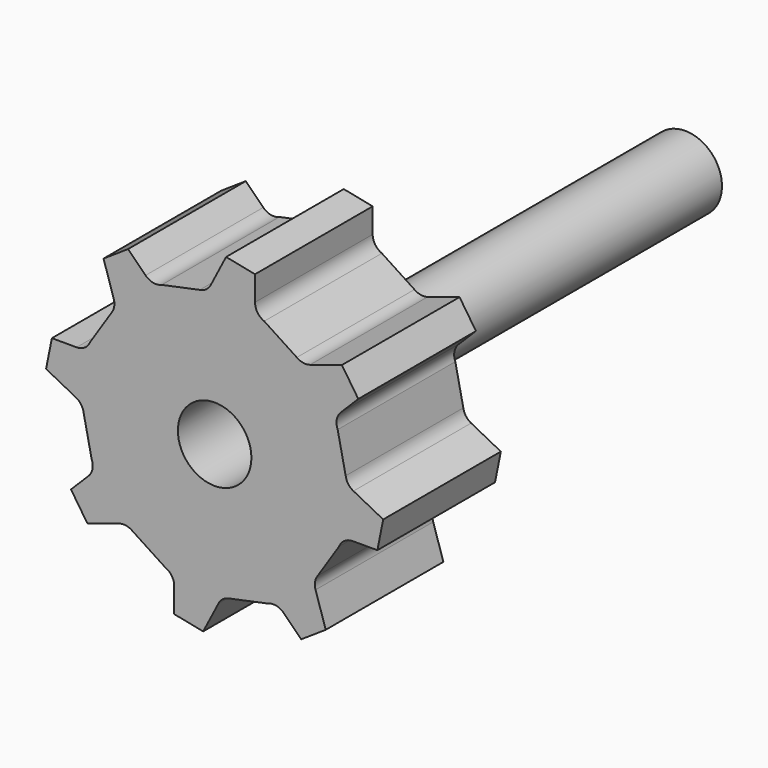
from build123d import *

# Parameters (mm, degrees)
F0_R     = 12.5
F1_DEPTH = 50
F2_R     = 12.5
F3_DEPTH = 150


with BuildPart() as f1:
    # F0 (on Front) → F1 (new body)
    with BuildSketch(Plane.XZ):
        with BuildLine():
            Line((-116.0371901115, -128.3445464136), (-125.8805584276, -126.3758683266))
            Line((-125.8805584276, -126.3758683266), (-131.1020102552, -136.4806844073))
            ThreePointArc((-131.1020102552, -136.4806844073), (-132.6345582421, -138.2516897117), (-134.8054626168, -139.1305169507))
            Line((-134.8054626168, -139.1305169507), (-147.7560899978, -141.8494963995))
            ThreePointArc((-147.7560899978, -141.8494963995), (-150.6647489323, -142.156192832), (-153.2473327671, -140.7833781193))
            Line((-153.2473327671, -140.7833781193), (-159.1905657596, -134.8401451268))
            Line((-159.1905657596, -134.8401451268), (-167.5429438709, -140.4083919875))
            Line((-167.5429438709, -140.4083919875), (-164.0898838925, -151.2456999557))
            ThreePointArc((-164.0898838925, -151.2456999557), (-163.9212691063, -153.5816648901), (-164.8349056108, -155.738150795))
            Line((-164.8349056108, -155.738150795), (-172.0697732464, -166.8182360428))
            ThreePointArc((-172.0697732464, -166.8182360428), (-173.9096385759, -169.0918356267), (-176.7065277112, -169.9472715767))
            Line((-176.7065277112, -169.9472715767), (-185.1115284135, -169.9472715767))
            Line((-185.1115284135, -169.9472715767), (-187.0802065005, -179.7906398927))
            Line((-187.0802065005, -179.7906398927), (-176.9753904198, -185.0120917203))
            ThreePointArc((-176.9753904198, -185.0120917203), (-175.2043851154, -186.5446397072), (-174.3255578764, -188.715544082))
            Line((-174.3255578764, -188.715544082), (-171.6065784276, -201.6661714629))
            ThreePointArc((-171.6065784276, -201.6661714629), (-171.2998819951, -204.5748303975), (-172.6726967078, -207.1574142323))
            Line((-172.6726967078, -207.1574142323), (-178.6159297003, -213.1006472248))
            Line((-178.6159297003, -213.1006472248), (-173.0476828396, -221.4530253361))
            Line((-173.0476828396, -221.4530253361), (-162.2103748713, -217.9999653577))
            ThreePointArc((-162.2103748713, -217.9999653577), (-159.874409937, -217.8313505714), (-157.7179240321, -218.7449870759))
            Line((-157.7179240321, -218.7449870759), (-146.6378387843, -225.9798547115))
            ThreePointArc((-146.6378387843, -225.9798547115), (-144.3642392004, -227.8197200411), (-143.5088032504, -230.6166091763))
            Line((-143.5088032504, -230.6166091763), (-143.5088032504, -239.0216098787))
            Line((-143.5088032504, -239.0216098787), (-133.6654349344, -240.9902879657))
            Line((-133.6654349344, -240.9902879657), (-128.4439831068, -230.8854718849))
            ThreePointArc((-128.4439831068, -230.8854718849), (-126.9114351199, -229.1144665805), (-124.7405307451, -228.2356393415))
            Line((-124.7405307451, -228.2356393415), (-111.7899033642, -225.5166598928))
            ThreePointArc((-111.7899033642, -225.5166598928), (-108.8812444296, -225.2099634602), (-106.2986605948, -226.5827781729))
            Line((-106.2986605948, -226.5827781729), (-100.3554276023, -232.5260111654))
            Line((-100.3554276023, -232.5260111654), (-92.003049491, -226.9577643047))
            Line((-92.003049491, -226.9577643047), (-95.4561094694, -216.1204563365))
            ThreePointArc((-95.4561094694, -216.1204563365), (-95.6247242557, -213.7844914022), (-94.7110877512, -211.6280054973))
            Line((-94.7110877512, -211.6280054973), (-87.4762201156, -200.5479202495))
            ThreePointArc((-87.4762201156, -200.5479202495), (-85.636354786, -198.2743206655), (-82.8394656508, -197.4188847156))
            Line((-82.8394656508, -197.4188847156), (-74.4344649484, -197.4188847156))
            Line((-74.4344649484, -197.4188847156), (-72.4657868614, -187.5755163995))
            Line((-72.4657868614, -187.5755163995), (-82.5706029422, -182.3540645719))
            ThreePointArc((-82.5706029422, -182.3540645719), (-84.3416082466, -180.821516585), (-85.2204354856, -178.6506122103))
            Line((-85.2204354856, -178.6506122103), (-87.9394149343, -165.6999848293))
            ThreePointArc((-87.9394149343, -165.6999848293), (-88.2461113669, -162.7913258948), (-86.8732966542, -160.20874206))
            Line((-86.8732966542, -160.20874206), (-80.9300636616, -154.2655090675))
            Line((-80.9300636616, -154.2655090675), (-86.4983105224, -145.9131309562))
            Line((-86.4983105224, -145.9131309562), (-97.3356184906, -149.3661909346))
            ThreePointArc((-97.3356184906, -149.3661909346), (-99.6715834249, -149.5348057208), (-101.8280693298, -148.6211692163))
            Line((-101.8280693298, -148.6211692163), (-112.9081545776, -141.3863015807))
            ThreePointArc((-112.9081545776, -141.3863015807), (-115.1817541616, -139.5464362512), (-116.0371901115, -136.7495471159))
            Line((-116.0371901115, -136.7495471159), (-116.0371901115, -128.3445464136))
        make_face()
        with Locations((-129.772996681, -183.6830781461)):
            Circle(F0_R, mode=Mode.SUBTRACT)
    extrude(amount=F1_DEPTH)


with BuildPart() as f3:
    # F2 (on face) → F3 (new body)
    with BuildSketch(Plane(origin=(0, 0, 0), x_dir=(-1, 0, 0), z_dir=(0, 1, 0))):
        with Locations((129.772996681, -183.6830781461)):
            Circle(F2_R)
    extrude(amount=F3_DEPTH)


solid = Compound([f1.part, f3.part])
